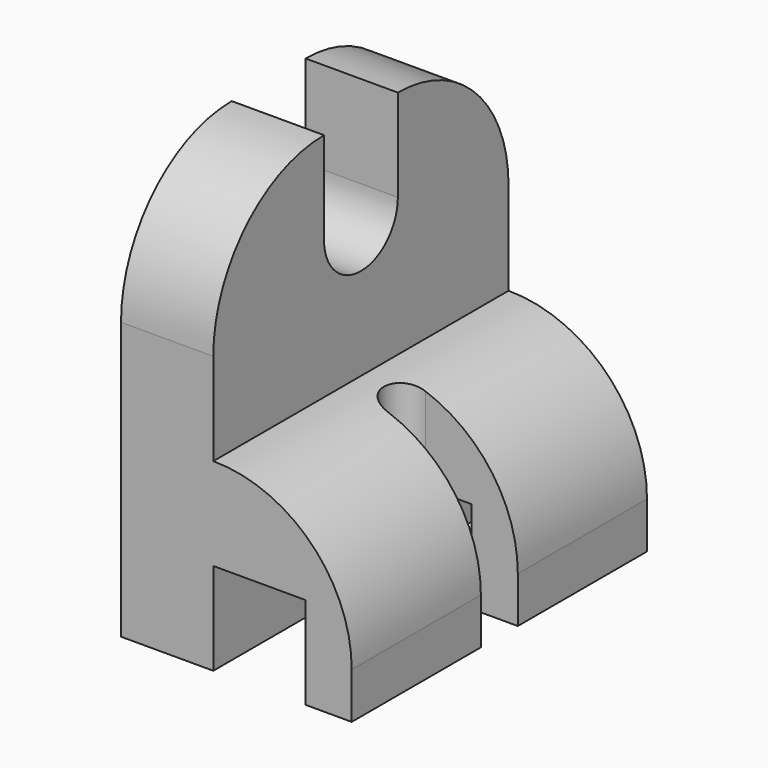
from build123d import *

# Parameters (mm, degrees)
F0_W      = 40
F0_H      = 20
F1_DEPTH  = 25
F2_W      = 10
F2_H      = 40
F3_DEPTH  = 25
F4_W      = 10
F4_H      = 2.6823076606
F5_DEPTH  = 50
F7_DEPTH  = 50
F8_R      = 14.99999
F9_F1_R   = 14.9999
F10_W     = 10
F10_H     = 10
F11_DEPTH = 100


# Not quite as in the source:
# - a fillet or chamfer is up to 0.001 mm smaller than in the source, because OpenCascade refuses the exact size


with BuildPart() as f1:
    # F0 (on Right) → F1 (new body)
    with BuildSketch(Plane.YZ):
        with Locations((20, 10)):
            Rectangle(F0_W, F0_H)
    extrude(amount=F1_DEPTH)

    # F2 (on face) → F3 (join)
    with BuildSketch(Plane.XY.offset(20)):
        with Locations((5, 20)):
            Rectangle(F2_W, F2_H)
    extrude(amount=F3_DEPTH)

    # F4 (on face) → F5 (cut)
    with BuildSketch(Plane.YZ.offset(10)):
        with BuildLine():
            Line((15, 45), (15, 35))
            ThreePointArc((15, 35), (20, 30), (25, 35))
            Line((25, 35), (25, 45))
            Line((25, 45), (15, 45))
        make_face()
        with Locations((20, 46.3411538303)):
            Rectangle(F4_W, F4_H)
    extrude(amount=-F5_DEPTH, mode=Mode.SUBTRACT)

    # F6 (on face) → F7 (cut)
    with BuildSketch(Plane.XY.offset(20)):
        with BuildLine():
            Line((25, 22.5), (15, 22.5))
            ThreePointArc((15, 22.5), (12.5, 20), (15, 17.5))
            Line((15, 17.5), (25, 17.5))
            Line((25, 17.5), (25, 22.5))
        make_face()
    extrude(amount=-F7_DEPTH, mode=Mode.SUBTRACT)

    # F8 (radius 15 in the source; OpenCascade refuses exactly that, so slightly less here)
    f8_edges = [f1.edges().sort_by_distance(p)[0] for p in [
        (5, 40, 45),
        (5, 0, 45),
    ]]
    fillet(f8_edges, radius=F8_R)

    # F9: fillet of radius 15 on 2 edges, made by hand

    # F9_f1 (radius 15 in the source; OpenCascade refuses exactly that, so slightly less here)
    f9_f1_edges = [f1.edges().sort_by_distance(p)[0] for p in [
        (25, 8.75, 20),
    ]]
    fillet(f9_f1_edges, radius=F9_F1_R)

    # F10 (on face) → F11 (cut)
    with BuildSketch(Plane(origin=(0, 40, 0), x_dir=(-1, 0, 0), z_dir=(0, 1, 0))):
        with Locations((-15, 5)):
            Rectangle(F10_W, F10_H)
    extrude(amount=-F11_DEPTH, mode=Mode.SUBTRACT)


solid = f1.part
